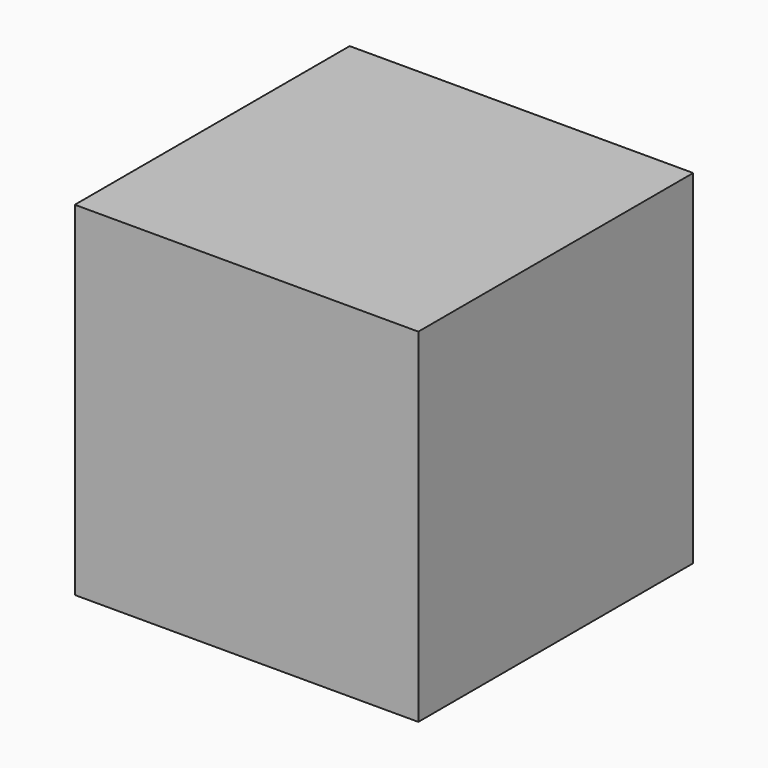
from build123d import *

# Parameters (mm, degrees)
F1_E0_W  = 25.3960397094
F1_E0_H  = 25.4
F2_DEPTH = 25.4


with BuildPart() as f2:
    # F1_E0 (on explicit) → F2 (new body)
    with BuildSketch(Plane(origin=(0, 0, 0), x_dir=(1, 0, 0), z_dir=(0, 0, -1))):
        with Locations((12.6980198547, 12.7)):
            Rectangle(F1_E0_W, F1_E0_H)
    extrude(amount=-F2_DEPTH)


solid = f2.part
